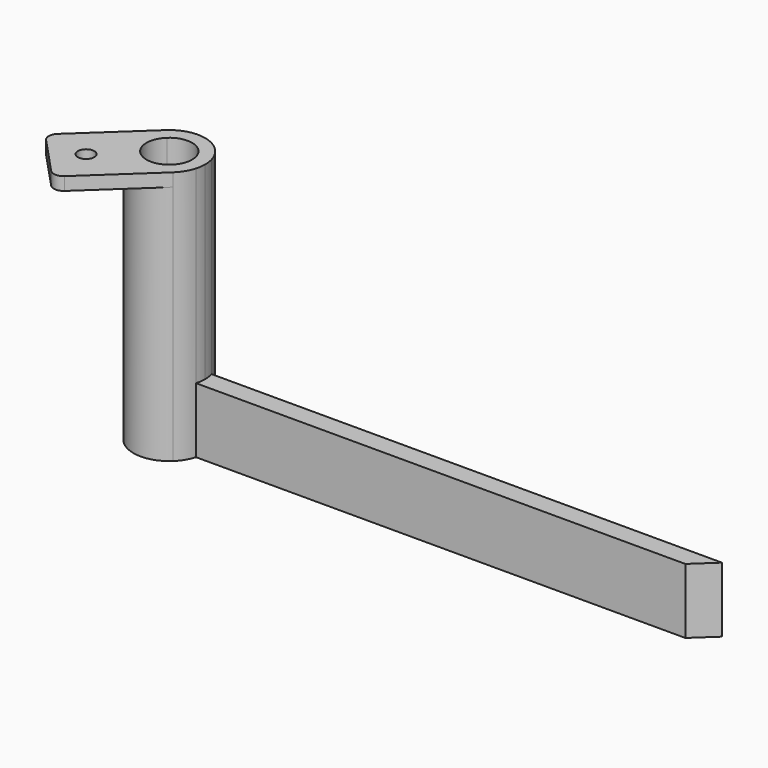
from build123d import *

# Parameters (mm, degrees)
F1_DEPTH = 10
F2_DEPTH = 39
F3_R     = 1.27
F4_DEPTH = 39
F0_R     = 1.27
F5_DEPTH = 37


# Not quite as in the source:
# - a feature names something its author has since deleted; it is built from what else it names


with BuildPart() as f1:
    # F0 (on Top) → F1 (new body)
    with BuildSketch(Plane.XY):
        with BuildLine():
            Line((39.0916730868, 1.5), (-39.2084973779, 1.5))
            ThreePointArc((-39.2084973779, 1.5), (-39.0523737086, 0.7572105316), (-39, 0))
            ThreePointArc((-39, 0), (-39.0523737086, -0.7572105316), (-39.2084973779, -1.5))
            Line((-39.2084973779, -1.5), (35.8745669567, -1.5))
            Line((35.8745669567, -1.5), (39.0916730868, 1.5))
        make_face()
    extrude(amount=F1_DEPTH)

    # F0 (on Top) → F2 (join)
    with BuildSketch(Plane.XY):
        with BuildLine():
            ThreePointArc((-42.1130057398, -2.5597379557), (-47.0597379557, -2.3869942602), (-46.8869942602, 2.5597379557))
            Line((-46.8869942602, 2.5597379557), (-48.2509909803, 4.0224453589))
            ThreePointArc((-48.2509909803, 4.0224453589), (-48.5224453589, -3.7509909803), (-40.7490090197, -4.0224453589))
            Line((-40.7490090197, -4.0224453589), (-42.1130057398, -2.5597379557))
        make_face()
        with BuildLine():
            ThreePointArc((-46.8869942602, 2.5597379557), (-43.1043782588, 3.2097102603), (-41, 0))
            ThreePointArc((-41, 0), (-41.2902897397, -1.3956217412), (-42.1130057398, -2.5597379557))
            Line((-42.1130057398, -2.5597379557), (-40.7490090197, -4.0224453589))
            ThreePointArc((-40.7490090197, -4.0224453589), (-39.8061364224, -2.866643458), (-39.2084973779, -1.5))
            ThreePointArc((-39.2084973779, -1.5), (-39.0523737086, -0.7572105316), (-39, 0))
            ThreePointArc((-39, 0), (-39.0523737086, 0.7572105316), (-39.2084973779, 1.5))
            ThreePointArc((-39.2084973779, 1.5), (-43.0221716349, 5.2977375665), (-48.2509909803, 4.0224453589))
            Line((-48.2509909803, 4.0224453589), (-46.8869942602, 2.5597379557))
        make_face()
    extrude(amount=F2_DEPTH)

    # F3 (on face) → F4 (join)
    with BuildSketch(Plane.XY):
        with BuildLine():
            Line((-50.2566071407, -12.8884240397), (-40.7490090197, -4.0224453589))
            ThreePointArc((-40.7490090197, -4.0224453589), (-48.5224453589, -3.7509909803), (-48.2509909803, 4.0224453589))
            Line((-48.2509909803, 4.0224453589), (-57.7585891014, -4.8435333219))
            ThreePointArc((-57.7585891014, -4.8435333219), (-58.2346778018, -5.8882146293), (-57.8326221137, -6.9635614144))
            Line((-57.8326221137, -6.9635614144), (-52.3766352332, -12.8143910274))
            ThreePointArc((-52.3766352332, -12.8143910274), (-51.3319539259, -13.2904797278), (-50.2566071407, -12.8884240397))
        make_face()
        with Locations((-51.8135370162, -6.8199836006)):
            Circle(F3_R, mode=Mode.SUBTRACT)
    extrude(amount=F4_DEPTH)

    # F0 (on Top) → F5 (cut)
    with BuildSketch(Plane.XY):
        with BuildLine():
            ThreePointArc((-40.7490090197, -4.0224453589), (-48.5224453589, -3.7509909803), (-48.2509909803, 4.0224453589))
            Line((-48.2509909803, 4.0224453589), (-57.7585891014, -4.8435333219))
            ThreePointArc((-57.7585891014, -4.8435333219), (-58.2346778018, -5.8882146293), (-57.8326221137, -6.9635614144))
            Line((-57.8326221137, -6.9635614144), (-52.3766352332, -12.8143910274))
            ThreePointArc((-52.3766352332, -12.8143910274), (-51.3319539259, -13.2904797278), (-50.2566071407, -12.8884240397))
            Line((-50.2566071407, -12.8884240397), (-40.7490090197, -4.0224453589))
        make_face()
        with Locations((-51.8135370162, -6.8199836006)):
            Circle(F0_R, mode=Mode.SUBTRACT)
    extrude(amount=F5_DEPTH, mode=Mode.SUBTRACT)


solid = f1.part
